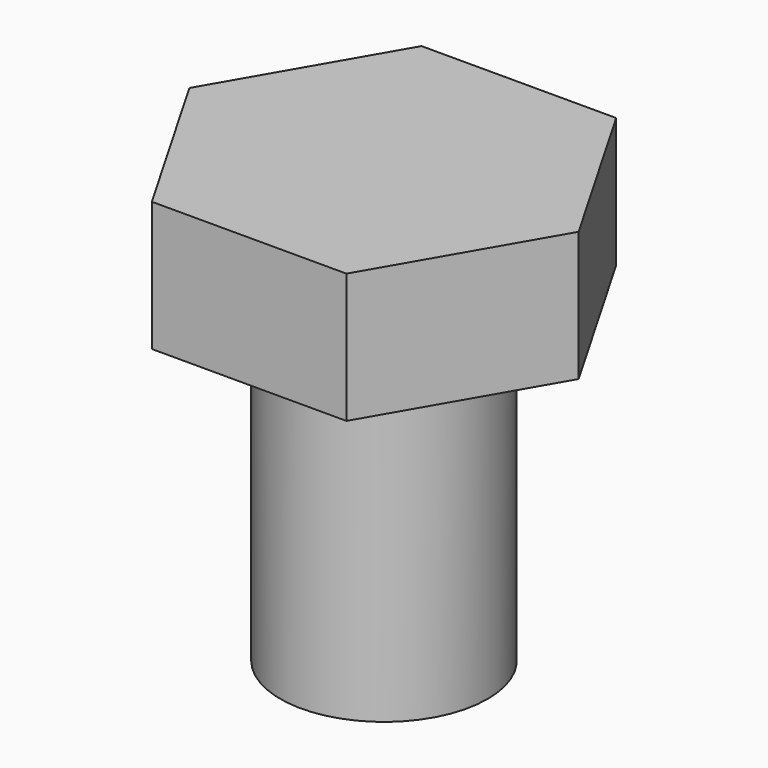
from build123d import *

# Parameters (mm, degrees)
F0_R     = 12.7
F1_DEPTH = 38.1
F3_DEPTH = 15.875


# Not quite as in the source:
# - a feature names something its author has since deleted; it is built from what else it names


with BuildPart() as f1:
    # F0 (on Top) → F1 (new body)
    with BuildSketch(Plane.XY):
        Circle(F0_R)
    extrude(amount=-F1_DEPTH)

    # F2 (on face) → F3 (join)
    with BuildSketch(Plane.XY):
        Polygon((11.9150661804, 20.6375), (-11.9150661804, 20.6375), (-23.8301323608, 0), (-11.9150661804, -20.6375), (11.9150661804, -20.6375), (23.8301323608, 0), align=None)
    extrude(amount=F3_DEPTH)


solid = f1.part
